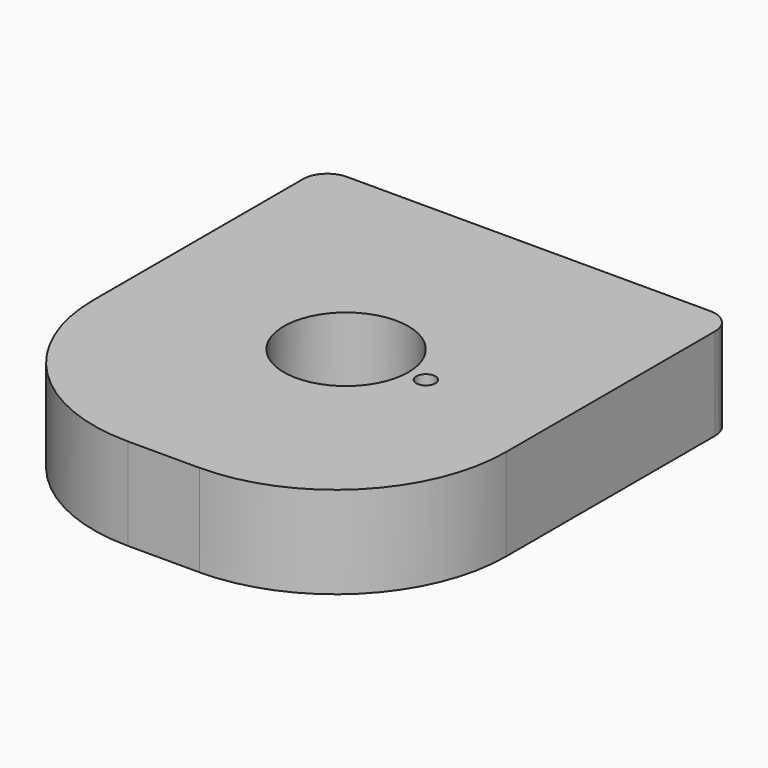
from build123d import *

# Parameters (mm, degrees)
F0_W     = 21.5
F0_H     = 23.8
F0_R     = 0.5
F0_R_2   = 3.25
F1_DEPTH = 4.8
F2_R     = 8.89
F3_R     = 1.27


# Not quite as in the source:
# - a feature of the source that left no trace in its solid (it failed there, or was rolled back) is left out


with BuildPart() as f1:
    # F0 (on Top) → F1 (new body)
    with BuildSketch(Plane.XY):
        with Locations((10.75, 11.9)):
            Rectangle(F0_W, F0_H)
        with Locations((14.9710876867, 11.8254814297)):
            Circle(F0_R, mode=Mode.SUBTRACT)
        with Locations((10.75, 11.9)):
            Circle(F0_R_2, mode=Mode.SUBTRACT)
    extrude(amount=F1_DEPTH)

    # F2
    f2_edges = [f1.edges().sort_by_distance(p)[0] for p in [
        (21.5, 0, 2.4),
        (0, 0, 2.4),
    ]]
    fillet(f2_edges, radius=F2_R)

    # F3
    f3_edges = [f1.edges().sort_by_distance(p)[0] for p in [
        (21.5, 23.8, 2.4),
        (0, 23.8, 2.4),
    ]]
    fillet(f3_edges, radius=F3_R)


solid = f1.part
